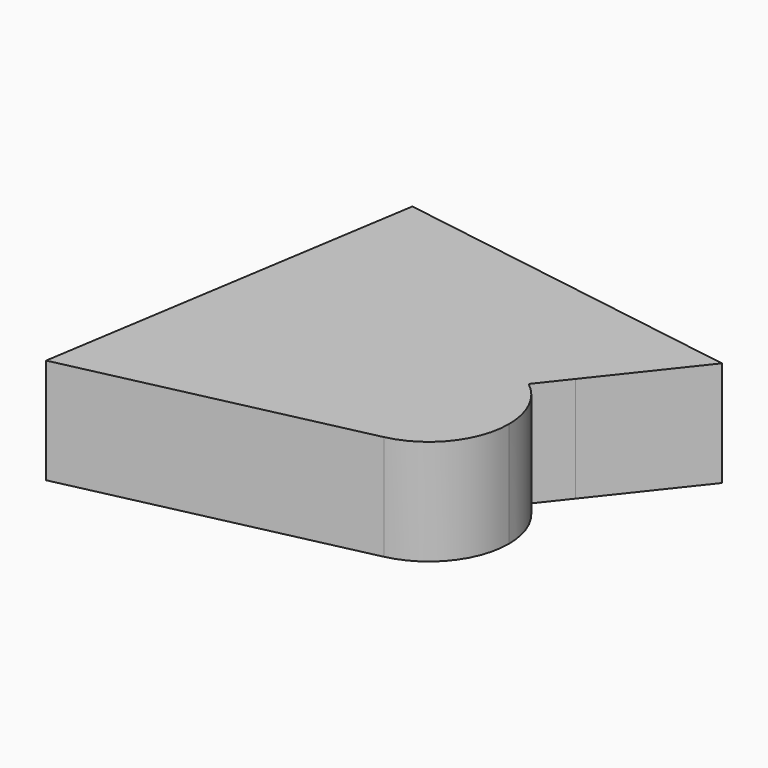
from build123d import *

# Parameters (mm, degrees)
F1_DEPTH = 25.4


# Not quite as in the source:
# - the program builds the solid bodies; features that only make, move or delete a surface that nothing else refers to are left out


with BuildPart() as f1:
    # F0 (on Top) → F1 (new body)
    with BuildSketch(Plane.XY):
        with BuildLine():
            ThreePointArc((19.282356954, 0), (17.3548102292, 8.4035618406), (11.957541655, 15.127011842))
            ThreePointArc((11.957541655, 15.127011842), (-18.7957142624, 4.3046968609), (4.1820366195, -18.823385971))
            ThreePointArc((4.1820366195, -18.823385971), (15.0407581689, -12.0658560991), (19.282356954, 0))
        make_face()
        with BuildLine():
            Line((11.957541655, 15.127011842), (17.5544340163, 22.2074184567))
            Line((17.5544340163, 22.2074184567), (35.1088680327, 44.4148369133))
            Line((35.1088680327, 44.4148369133), (-50.3368154168, 57.9507872462))
            Line((-50.3368154168, 57.9507872462), (-64.9315572131, -34.1785170794))
            Line((-64.9315572131, -34.1785170794), (4.1820366195, -18.823385971))
            ThreePointArc((4.1820366195, -18.823385971), (-18.7957142624, 4.3046968609), (11.957541655, 15.127011842))
        make_face()
    extrude(amount=F1_DEPTH)


solid = f1.part
